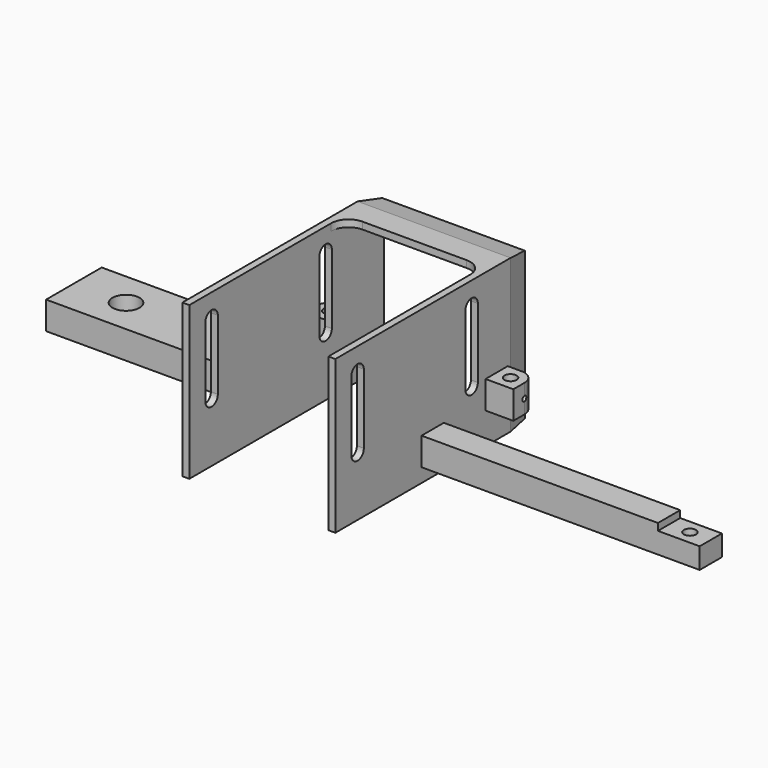
from build123d import *

# Parameters (mm, degrees)
F0_W         = 44
F0_H         = 44
F1_DEPTH     = 70
F2_W         = 40
F2_H         = 42
F3_DEPTH     = 70
F5_DEPTH     = 44
F7_DEPTH     = 2
F9_W         = 8
F9_H         = 8
F10_DEPTH    = 80
F11_W        = 8
F11_H        = 2
F12_DEPTH    = 12
F13_W        = 20
F13_H        = 8
F14_DEPTH    = 50
F15_W        = 15
F15_H        = 2
F16_DEPTH    = 50
F17_R        = 3.9
F18_DEPTH    = 20
F19_SIZE2    = 1.5
F19_SIZE     = 7
F20_SIZE2    = 7
F20_SIZE     = 1.5
F21_SIZE2    = 7
F21_SIZE     = 1.5
F22_R        = 1.75
F23_DEPTH    = 8
F24_DEPTH    = 44
F25_W        = 8
F25_H        = 8
F25_R        = 0.75
F26_DEPTH    = 8
F27_R        = 1.75
F28_DEPTH    = 8
F29_T1_DEPTH = 28
F30_W        = 8
F30_H        = 8
F30_R        = 0.75
F31_DEPTH    = 8
F32_R        = 1.75
F33_DEPTH    = 8
F34_T1_DEPTH = 28


# Not quite as in the source:
# - a fillet or chamfer that OpenCascade refuses, or shapes differently, is made with other operations: its cross-section is extruded or revolved along the edge and cut away or added


with BuildPart() as f1:
    # F0 (on Front) → F1 (new body)
    with BuildSketch(Plane.XZ):
        with Locations((22, 22)):
            Rectangle(F0_W, F0_H)
    extrude(amount=-F1_DEPTH)

    # F2 (on face) → F3 (cut, through all)
    with BuildSketch(Plane.XZ):
        with Locations((22, 21)):
            Rectangle(F2_W, F2_H)
    extrude(amount=-F3_DEPTH, mode=Mode.SUBTRACT)

    # F4 (on face) → F5 (cut)
    with BuildSketch(Plane.YZ.offset(44)):
        with BuildLine():
            ThreePointArc((51.25, 37.25), (49, 39.5), (46.75, 37.25))
            Line((46.75, 37.25), (46.75, 17.25))
            ThreePointArc((46.75, 17.25), (49, 15), (51.25, 17.25))
            Line((51.25, 17.25), (51.25, 37.25))
        make_face()
    extrude(amount=-F5_DEPTH, mode=Mode.SUBTRACT)

    # F6 (on face) → F7 (cut, through all)
    with BuildSketch(Plane.XY.offset(44)):
        with BuildLine():
            Line((2, 51), (2, 0))
            Line((2, 0), (42, 0))
            Line((42, 0), (42, 51))
            ThreePointArc((42, 51), (40.5355339059, 54.5355339059), (37, 56))
            Line((37, 56), (7, 56))
            ThreePointArc((7, 56), (3.4644660941, 54.5355339059), (2, 51))
        make_face()
    extrude(amount=-F7_DEPTH, mode=Mode.SUBTRACT)

    # F9 (on face) → F10 (join)
    with BuildSketch(Plane.YZ.offset(44)):
        with Locations((35, 8)):
            Rectangle(F9_W, F9_H)
    extrude(amount=F10_DEPTH)

    # F11 (on face) → F12 (cut)
    with BuildSketch(Plane.YZ.offset(124)):
        with Locations((35, 11)):
            Rectangle(F11_W, F11_H)
    extrude(amount=-F12_DEPTH, mode=Mode.SUBTRACT)

    # F13 (on face) → F14 (join)
    with BuildSketch(Plane(origin=(0, 0, 0), x_dir=(0, -1, 0), z_dir=(-1, 0, 0))):
        with Locations((-23.5, 19)):
            Rectangle(F13_W, F13_H)
    extrude(amount=F14_DEPTH)

    # F15 (on face) → F16 (cut, through all)
    with BuildSketch(Plane(origin=(-50, 0, 0), x_dir=(0, -1, 0), z_dir=(-1, 0, 0))):
        with Locations((-23.5, 16)):
            Rectangle(F15_W, F15_H)
    extrude(amount=-F16_DEPTH, mode=Mode.SUBTRACT)

    # F17 (on face) → F18 (cut)
    with BuildSketch(Plane.XY.offset(23)):
        with Locations((-35, 23.5)):
            Circle(F17_R)
    extrude(amount=-F18_DEPTH, mode=Mode.SUBTRACT)

    # F19
    f19_edges = [f1.edges().sort_by_distance(p)[0] for p in [
        (44, 70, 22),
    ]]
    f19_side = f1.faces().sort_by_distance((44, 34.490511, 22.116835))[0]
    chamfer(f19_edges, length=F19_SIZE, length2=F19_SIZE2, reference=f19_side)

    # F20
    f20_edges = [f1.edges().sort_by_distance(p)[0] for p in [
        (21.25, 70, 44),
    ]]
    f20_side = f1.faces().sort_by_distance((21.25, 70, 43.388261))[0]
    chamfer(f20_edges, length=F20_SIZE, length2=F20_SIZE2, reference=f20_side)

    # F21
    f21_edges = [f1.edges().sort_by_distance(p)[0] for p in [
        (0, 70, 21.25),
    ]]
    f21_side = f1.faces().sort_by_distance((42.439896, 70, 21.25))[0]
    chamfer(f21_edges, length=F21_SIZE, length2=F21_SIZE2, reference=f21_side)

    # F22 (on face) → F23 (cut)
    with BuildSketch(Plane.XY.offset(10)):
        with Locations((118, 35)):
            Circle(F22_R)
    extrude(amount=-F23_DEPTH, mode=Mode.SUBTRACT)

    # F8 (on face) → F24 (cut)
    with BuildSketch(Plane.YZ.offset(44)):
        with BuildLine():
            ThreePointArc((10.25, 37.25), (8, 39.5), (5.75, 37.25))
            Line((5.75, 37.25), (5.75, 17.25))
            ThreePointArc((5.75, 17.25), (8, 15), (10.25, 17.25))
            Line((10.25, 17.25), (10.25, 37.25))
        make_face()
    extrude(amount=-F24_DEPTH, mode=Mode.SUBTRACT)

    # F25 (on face) → F26 (join)
    with BuildSketch(Plane.YZ.offset(44)):
        with Locations((58, 13)):
            Rectangle(F25_W, F25_H)
        with Locations((58, 13)):
            Circle(F25_R, mode=Mode.SUBTRACT)
    extrude(amount=F26_DEPTH)

    # F27 (on face) → F28 (cut)
    with BuildSketch(Plane.XY.offset(17)):
        with Locations((48, 58)):
            Circle(F27_R)
    extrude(amount=-F28_DEPTH, mode=Mode.SUBTRACT)

    # F29: fillet of radius 4 on 1 edges, made by hand

    # F29_s2 → F29_t1 (cut)
    with BuildSketch(Plane.XY.offset(-1)):
        with BuildLine():
            ThreePointArc((48, 62), (50.8284271247, 60.8284271247), (52, 58))
            Line((52, 58), (52, 62))
            Line((52, 62), (48, 62))
        make_face()
    extrude(amount=F29_T1_DEPTH, mode=Mode.SUBTRACT)

    # F30 (on face) → F31 (join)
    with BuildSketch(Plane(origin=(0, 0, 0), x_dir=(0, -1, 0), z_dir=(-1, 0, 0))):
        with Locations((-58, 13)):
            Rectangle(F30_W, F30_H)
        with Locations((-58, 13)):
            Circle(F30_R, mode=Mode.SUBTRACT)
    extrude(amount=F31_DEPTH)

    # F32 (on face) → F33 (cut)
    with BuildSketch(Plane.XY.offset(17)):
        with Locations((-4, 58)):
            Circle(F32_R)
    extrude(amount=-F33_DEPTH, mode=Mode.SUBTRACT)

    # F34: fillet of radius 4 on 1 edges, made by hand

    # F34_s2 → F34_t1 (cut)
    with BuildSketch(Plane.XY.offset(-1)):
        with BuildLine():
            ThreePointArc((-4, 62), (-6.8284271247, 60.8284271247), (-8, 58))
            Line((-8, 58), (-8, 62))
            Line((-8, 62), (-4, 62))
        make_face()
    extrude(amount=F34_T1_DEPTH, mode=Mode.SUBTRACT)


solid = f1.part
